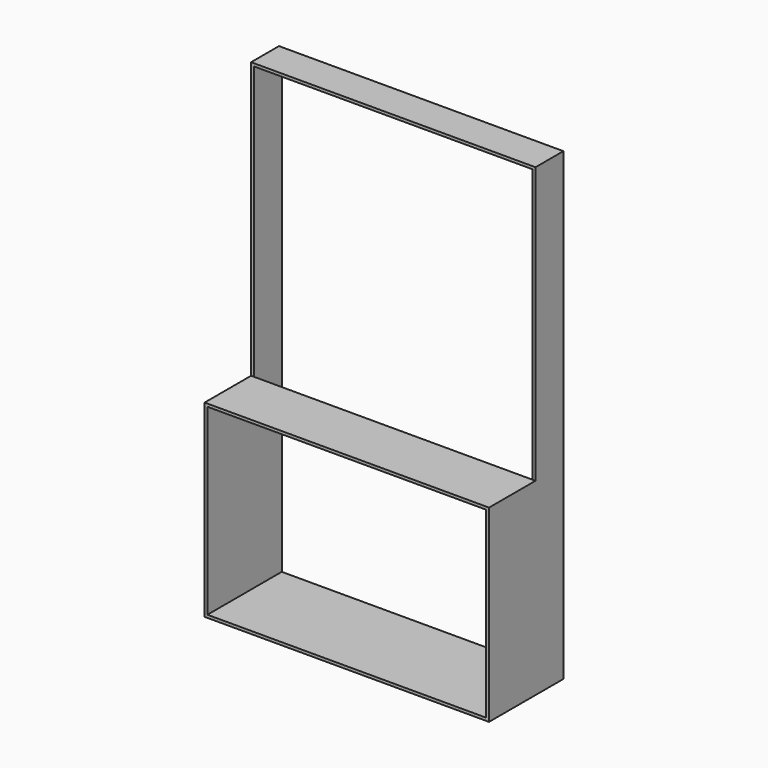
from build123d import *

# Parameters (mm, degrees)
F0_W     = 1224
F0_H     = 400
F1_DEPTH = 2000
F2_W     = 1224
F2_H     = 1188
F3_DEPTH = 250
F4_T     = -12


# Not quite as in the source:
# - a shell that OpenCascade refuses in one call is made with other operations: the cavity is built on its own and cut out


with BuildPart() as f1:
    # F0 (on Top) → F1 (new body)
    with BuildSketch(Plane.XY):
        Rectangle(F0_W, F0_H)
    extrude(amount=F1_DEPTH)

    # F2 (on face) → F3 (cut)
    with BuildSketch(Plane.XZ.offset(200)):
        with Locations((0, 1406)):
            Rectangle(F2_W, F2_H)
    extrude(amount=-F3_DEPTH, mode=Mode.SUBTRACT)

    # F4: a shell. OpenCascade refuses it in one call, so the cavity is built on its own and cut out:
    # the body offset inwards by the wall thickness, plus a prism from it out through each open face.
    f4_core = offset(f1.part, amount=F4_T, kind=Kind.INTERSECTION, mode=Mode.PRIVATE)
    f4_exits = [f4_core.faces().sort_by_distance(p)[0] for p in [
        (0, 188, 1000),
        (0, 62, 1394),
        (0, -188, 406),
    ]]
    add(f4_core, mode=Mode.SUBTRACT)
    extrude(f4_exits, amount=-F4_T, mode=Mode.SUBTRACT)


solid = f1.part
